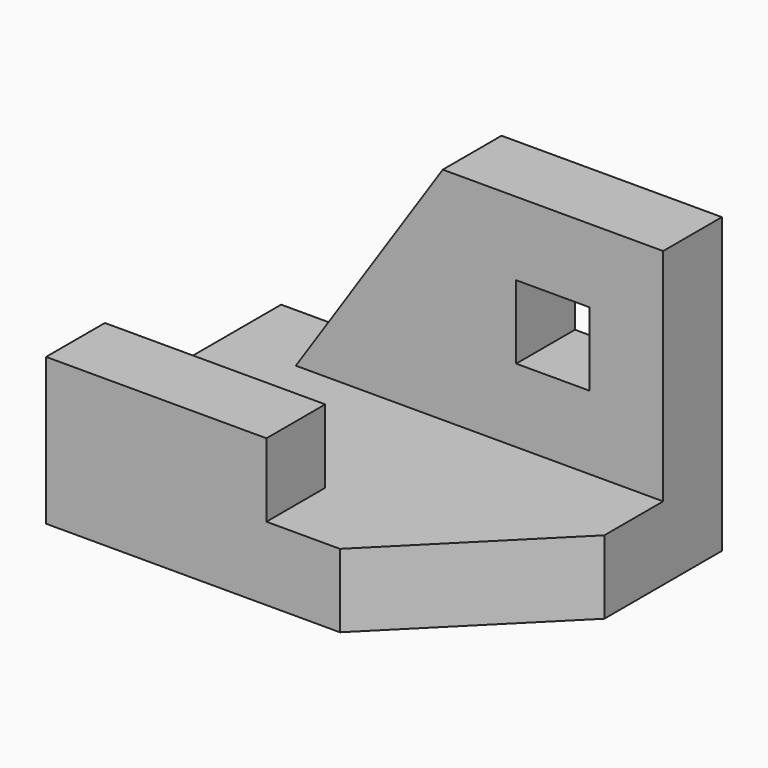
from build123d import *

# Parameters (mm, degrees)
F0_W     = 30
F0_H     = 10
F0_W_2   = 50
F1_DEPTH = 10
F2_DEPTH = 10
F3_DEPTH = 30
F4_W     = 10
F4_H     = 10
F5_DEPTH = 10
F6_SIZE2 = 29.99999
F6_SIZE  = 19.99999


# Not quite as in the source:
# - a fillet or chamfer is up to 0.001 mm smaller than in the source, because OpenCascade refuses the exact size


with BuildPart() as f1:
    # F0 (on Top) → F1 (new body)
    with BuildSketch(Plane.XY):
        with Locations((15, 5)):
            Rectangle(F0_W, F0_H)
        with Locations((35, 35)):
            Rectangle(F0_W_2, F0_H)
        Polygon((30, 10), (30, 0), (40, 0), (60, 20), (60, 30), (10, 30), (10, 40), (0, 40), (0, 10), align=None)
    extrude(amount=-F1_DEPTH)

    # F0 (on Top) → F2 (join)
    with BuildSketch(Plane.XY):
        with Locations((15, 5)):
            Rectangle(F0_W, F0_H)
    extrude(amount=F2_DEPTH)

    # F0 (on Top) → F3 (join)
    with BuildSketch(Plane.XY):
        with Locations((35, 35)):
            Rectangle(F0_W_2, F0_H)
    extrude(amount=F3_DEPTH)

    # F4 (on face) → F5 (cut)
    with BuildSketch(Plane(origin=(0, 40, 0), x_dir=(-1, 0, 0), z_dir=(0, 1, 0))):
        with Locations((-45, 15)):
            Rectangle(F4_W, F4_H)
    extrude(amount=-F5_DEPTH, mode=Mode.SUBTRACT)

    # F6 (size 20 and 30 in the source; OpenCascade refuses exactly that, so slightly less here)
    f6_edges = [f1.edges().sort_by_distance(p)[0] for p in [
        (10, 35, 30),
    ]]
    f6_side = f1.faces().sort_by_distance((35, 35, 30))[0]
    chamfer(f6_edges, length=F6_SIZE, length2=F6_SIZE2, reference=f6_side)


solid = f1.part
